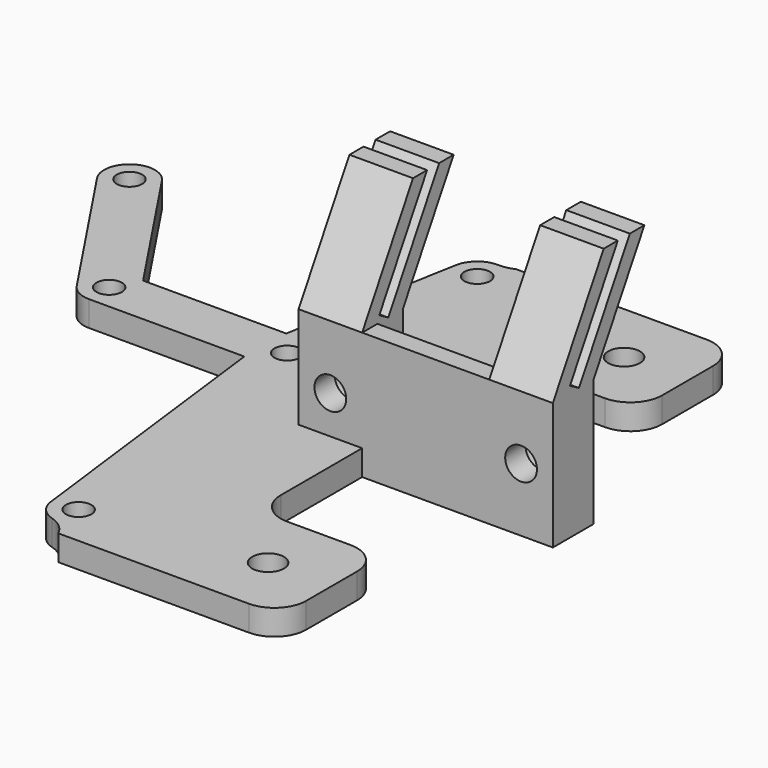
from build123d import *

# Parameters (mm, degrees)
F0_W         = 20
F0_H         = 4
F1_DEPTH     = 20
F2_DEPTH     = 20
F4_START     = 10
F4_DEPTH     = 10
F5_START     = -10
F5_DEPTH     = 10
F6_R         = 2.5
F7_DEPTH     = 25
F6_R_2       = 4.25
F8_DEPTH     = 4
F9_DEPTH     = 1
F10_W        = 20
F10_H        = 20
F10_R        = 2.5
F10_R_2      = 2
F11_DEPTH    = 4
F12_T1_DEPTH = 4
F13_R        = 5


# Not quite as in the source:
# - a fillet or chamfer that OpenCascade refuses, or shapes differently, is made with other operations: its cross-section is extruded or revolved along the edge and cut away or added
# - ends of sketch curves that miss each other by under 0.0002 mm in the source are joined


with BuildPart() as f1:
    # F0 (on Top) → F1 (new body)
    with BuildSketch(Plane.XY):
        with Locations((0, -2)):
            Rectangle(F0_W, F0_H)
    extrude(amount=F1_DEPTH)

    # F0 (on Top) → F2 (join)
    with BuildSketch(Plane.XY):
        Polygon((-10, 4), (-20, 4), (-20, -4), (-10, -4), (-10, 0), align=None)
        Polygon((20, 4), (10, 4), (10, 0), (10, -4), (20, -4), align=None)
    extrude(amount=F2_DEPTH)

    # F3 (on Right) → F4 (join)
    with BuildSketch(Plane.YZ.offset(F4_START)):
        Polygon((-4, 20), (-1.2287187079, 20), (-0.636934682, 21.025), (8.7712812921, 37.3205080757), (6, 37.3205080757), align=None)
        Polygon((-1.2287187079, 20), (1.1384173958, 20), (-0.636934682, 21.025), align=None)
        Polygon((1.1384173958, 20), (4, 20), (14, 37.3205080757), (11.1384173958, 37.3205080757), align=None)
    extrude(amount=F4_DEPTH)

    # F3 (on Right) → F5 (join)
    with BuildSketch(Plane.YZ.offset(F5_START)):
        Polygon((1.1384173958, 20), (4, 20), (14, 37.3205080757), (11.1384173958, 37.3205080757), align=None)
        Polygon((-4, 20), (-1.2287187079, 20), (-0.636934682, 21.025), (8.7712812921, 37.3205080757), (6, 37.3205080757), align=None)
        Polygon((-1.2287187079, 20), (1.1384173958, 20), (-0.636934682, 21.025), align=None)
    extrude(amount=-F5_DEPTH)

    # F6 (on face) → F7 (cut)
    with BuildSketch(Plane(origin=(0, 4, 0), x_dir=(-1, 0, 0), z_dir=(0, 1, 0))):
        with Locations((-15, 10)):
            Circle(F6_R)
        with Locations((15, 10)):
            Circle(F6_R)
    extrude(amount=-F7_DEPTH, mode=Mode.SUBTRACT)

    # F6 (on face) → F8 (cut)
    with BuildSketch(Plane(origin=(0, 4, 0), x_dir=(-1, 0, 0), z_dir=(0, 1, 0))):
        with Locations((-15, 10)):
            Circle(F6_R_2)
        with Locations((-15, 10)):
            Circle(F6_R, mode=Mode.SUBTRACT)
        with Locations((15, 10)):
            Circle(F6_R_2)
        with Locations((15, 10)):
            Circle(F6_R, mode=Mode.SUBTRACT)
    extrude(amount=-F8_DEPTH, mode=Mode.SUBTRACT)

    # F9 (cut): a face of the model
    f9_faces = [f1.faces().sort_by_distance(p)[0] for p in [
        (0, 0, 10),
    ]]
    extrude(f9_faces, amount=-F9_DEPTH, mode=Mode.SUBTRACT)


with BuildPart() as f11:
    # F10 (on Top) → F11 (new body)
    with BuildSketch(Plane.XY):
        with Locations((0, 35)):
            Rectangle(F10_W, F10_H)
        with Locations((0, 35)):
            Circle(F10_R, mode=Mode.SUBTRACT)
        with BuildLine():
            Line((-10, 25), (-10, 45))
            Line((-10, 45), (-25, 45))
            Line((-25, 45), (-25, 44.5))
            Line((-25, 44.5), (-25, 43.6224989992))
            ThreePointArc((-25, 43.6224989992), (-23.8944487245, 42.2320508076), (-23.5, 40.5))
            ThreePointArc((-23.5, 40.5), (-23.5159046021, 40.1436520514), (-23.5634919302, 39.7901378891))
            Line((-23.5634919302, 39.7901378891), (-25, 31.8240476839))
            Line((-25, 31.8240476839), (-25, 14))
            Line((-25, 14), (-25, 6))
            Line((-25, 6), (-25, -22.0868501472))
            Line((-25, -22.0868501472), (-23.0302620717, -38.0088984006))
            ThreePointArc((-23.0302620717, -38.0088984006), (-23.0075726861, -38.2539834488), (-23, -38.5))
            ThreePointArc((-23, -38.5), (-23.5358983849, -40.5), (-25, -41.9641016151))
            Line((-25, -41.9641016151), (-25, -42.5))
            Line((-25, -42.5), (-25, -45))
            Line((-25, -45), (-10, -45))
            Line((-10, -45), (-10, -25))
            Line((-10, -25), (-10, 25))
        make_face()
        with Locations((0, -35)):
            Rectangle(F10_W, F10_H)
        with Locations((0, -35)):
            Circle(F10_R, mode=Mode.SUBTRACT)
        with BuildLine():
            Line((-36.5356474045, 6), (-30.9697379283, -38.9911015994))
            ThreePointArc((-30.9697379283, -38.9911015994), (-29.9970323987, -35.8508875446), (-27, -34.5))
            Line((-27, -34.5), (-25, -34.5))
            Line((-25, -34.5), (-25, -22.0868501472))
            Line((-25, -22.0868501472), (-28.4746618739, 6))
            Line((-28.4746618739, 6), (-33, 6))
            Line((-33, 6), (-36.5356474045, 6))
        make_face()
        Polygon((-25, 6), (-25, 14), (-28.2141725332, 14), (-28.9556634317, 9.8880959261), (-28.4746618739, 6), align=None)
        with BuildLine():
            Line((-25, -34.5), (-25, -35.0358983849))
            ThreePointArc((-25, -35.0358983849), (-23.665464799, -36.29072976), (-23.0302620717, -38.0088984006))
            Line((-23.0302620717, -38.0088984006), (-25, -22.0868501472))
            Line((-25, -22.0868501472), (-25, -34.5))
        make_face()
        with BuildLine():
            ThreePointArc((-27, -34.5), (-25.9647238196, -34.6362966948), (-25, -35.0358983849))
            Line((-25, -35.0358983849), (-25, -34.5))
            Line((-25, -34.5), (-27, -34.5))
        make_face()
        with BuildLine():
            Line((-25, -38.5), (-25, -41.9641016151))
            ThreePointArc((-25, -41.9641016151), (-23.5358983849, -40.5), (-23, -38.5))
            ThreePointArc((-23, -38.5), (-23.0075726861, -38.2539834488), (-23.0302620717, -38.0088984006))
            ThreePointArc((-23.0302620717, -38.0088984006), (-23.665464799, -36.29072976), (-25, -35.0358983849))
            Line((-25, -35.0358983849), (-25, -38.5))
        make_face()
        with BuildLine():
            ThreePointArc((-27, -42.5), (-25.9647238196, -42.3637033052), (-25, -41.9641016151))
            Line((-25, -41.9641016151), (-25, -38.5))
            Line((-25, -38.5), (-25, -35.0358983849))
            ThreePointArc((-25, -35.0358983849), (-25.9647238196, -34.6362966948), (-27, -34.5))
            ThreePointArc((-27, -34.5), (-29.9970323987, -35.8508875446), (-30.9697379283, -38.9911015994))
            ThreePointArc((-30.9697379283, -38.9911015994), (-29.6491124554, -41.4970323987), (-27, -42.5))
        make_face()
        with Locations((-27, -38.5)):
            Circle(F10_R_2, mode=Mode.SUBTRACT)
        with BuildLine():
            Line((-27, -42.5), (-25, -42.5))
            Line((-25, -42.5), (-25, -41.9641016151))
            ThreePointArc((-25, -41.9641016151), (-25.9647238196, -42.3637033052), (-27, -42.5))
        make_face()
        Polygon((-25, -22.0868501472), (-25, 6), (-28.4746618739, 6), align=None)
        Polygon((-25, 14), (-25, 31.8240476839), (-28.2141725332, 14), align=None)
        with BuildLine():
            Line((-28.4746618739, 6), (-28.9556634317, 9.8880959261))
            Line((-28.9556634317, 9.8880959261), (-29.0634919302, 9.2901378891))
            ThreePointArc((-29.0634919302, 9.2901378891), (-30.4347951781, 6.9308430764), (-33, 6))
            Line((-33, 6), (-28.4746618739, 6))
        make_face()
        with BuildLine():
            ThreePointArc((-33, 6), (-35.6491124554, 7.0029676013), (-36.9697379283, 9.5088984006))
            Line((-36.9697379283, 9.5088984006), (-36.5356474045, 6))
            Line((-36.5356474045, 6), (-33, 6))
        make_face()
        with BuildLine():
            Line((-33, 14), (-36.3432041846, 14))
            Line((-36.3432041846, 14), (-36.9365077488, 10.7098620531))
            ThreePointArc((-36.9365077488, 10.7098620531), (-35.5652048219, 13.0691569236), (-33, 14))
        make_face()
        with BuildLine():
            Line((-28.2141725332, 14), (-33, 14))
            ThreePointArc((-33, 14), (-30.3508875446, 12.9970323987), (-29.0302620717, 10.4911015994))
            Line((-29.0302620717, 10.4911015994), (-28.9556634317, 9.8880959261))
            Line((-28.9556634317, 9.8880959261), (-28.2141725332, 14))
        make_face()
        with BuildLine():
            ThreePointArc((-27.5, 36.5), (-30.5691569236, 37.9347951781), (-31.4365080698, 41.2098621109))
            Line((-31.4365080698, 41.2098621109), (-36.3432041846, 14))
            Line((-36.3432041846, 14), (-33, 14))
            Line((-33, 14), (-28.2141725332, 14))
            Line((-28.2141725332, 14), (-25, 31.8240476839))
            Line((-25, 31.8240476839), (-25, 36.5))
            Line((-25, 36.5), (-27.5, 36.5))
        make_face()
        with BuildLine():
            ThreePointArc((-23.5634919302, 39.7901378891), (-24.0630881272, 38.4536283871), (-25, 37.3775010008))
            Line((-25, 37.3775010008), (-25, 36.5))
            Line((-25, 36.5), (-25, 31.8240476839))
            Line((-25, 31.8240476839), (-23.5634919302, 39.7901378891))
        make_face()
        with BuildLine():
            Line((-25, 36.5), (-25, 37.3775010008))
            ThreePointArc((-25, 37.3775010008), (-26.1752351146, 36.7257453718), (-27.5, 36.5))
            Line((-27.5, 36.5), (-25, 36.5))
        make_face()
        with BuildLine():
            Line((-25, 37.3775010008), (-25, 43.6224989992))
            ThreePointArc((-25, 43.6224989992), (-26.1752351146, 44.2742546282), (-27.5, 44.5))
            ThreePointArc((-27.5, 44.5), (-30.0652048219, 43.5691569236), (-31.4365080698, 41.2098621109))
            ThreePointArc((-31.4365080698, 41.2098621109), (-30.5691569236, 37.9347951781), (-27.5, 36.5))
            ThreePointArc((-27.5, 36.5), (-26.1752351146, 36.7257453718), (-25, 37.3775010008))
        make_face()
        with Locations((-27.5, 40.5)):
            Circle(F10_R_2, mode=Mode.SUBTRACT)
        with BuildLine():
            ThreePointArc((-23.5, 40.5), (-23.8944487245, 42.2320508076), (-25, 43.6224989992))
            Line((-25, 43.6224989992), (-25, 37.3775010008))
            ThreePointArc((-25, 37.3775010008), (-24.0630881272, 38.4536283871), (-23.5634919302, 39.7901378891))
            ThreePointArc((-23.5634919302, 39.7901378891), (-23.5159046021, 40.1436520514), (-23.5, 40.5))
        make_face()
        with BuildLine():
            Line((-25, 43.6224989992), (-25, 44.5))
            Line((-25, 44.5), (-27.5, 44.5))
            ThreePointArc((-27.5, 44.5), (-26.1752351146, 44.2742546282), (-25, 43.6224989992))
        make_face()
        with BuildLine():
            Line((-36.9365077488, 10.7098620531), (-36.3432041846, 14))
            Line((-36.3432041846, 14), (-58.859264966, 14))
            Line((-58.859264966, 14), (-57.6717988226, 12.2188007849))
            ThreePointArc((-57.6717988226, 12.2188007849), (-57.171631894, 11.1591365948), (-57, 10))
            ThreePointArc((-57, 10), (-58.1715728753, 7.1715728753), (-61, 6))
            Line((-61, 6), (-36.5356474045, 6))
            Line((-36.5356474045, 6), (-36.9697379283, 9.5088984006))
            ThreePointArc((-36.9697379283, 9.5088984006), (-36.9984696952, 10.1106349684), (-36.9365077488, 10.7098620531))
        make_face()
        with BuildLine():
            ThreePointArc((-57, 10), (-57.171631894, 11.1591365948), (-57.6717988226, 12.2188007849))
            ThreePointArc((-57.6717988226, 12.2188007849), (-59.1125682979, 13.5266983951), (-61, 14))
            ThreePointArc((-61, 14), (-64.5266983951, 11.8874317021), (-64.3282011774, 7.7811992151))
            ThreePointArc((-64.3282011774, 7.7811992151), (-62.8874317021, 6.4733016049), (-61, 6))
            ThreePointArc((-61, 6), (-58.1715728753, 7.1715728753), (-57, 10))
        make_face()
        with Locations((-61, 10)):
            Circle(F10_R_2, mode=Mode.SUBTRACT)
        with BuildLine():
            Line((-57.6717988226, 12.2188007849), (-58.859264966, 14))
            Line((-58.859264966, 14), (-61, 14))
            ThreePointArc((-61, 14), (-59.1125682979, 13.5266983951), (-57.6717988226, 12.2188007849))
        make_face()
        with BuildLine():
            Line((-61, 14), (-58.859264966, 14))
            Line((-58.859264966, 14), (-73.6717988226, 36.2188007849))
            ThreePointArc((-73.6717988226, 36.2188007849), (-73.171631894, 35.1591365948), (-73, 34))
            ThreePointArc((-73, 34), (-75.8408634052, 30.171631894), (-80.3282011774, 31.7811992151))
            Line((-80.3282011774, 31.7811992151), (-64.3282011774, 7.7811992151))
            ThreePointArc((-64.3282011774, 7.7811992151), (-64.5266983951, 11.8874317021), (-61, 14))
        make_face()
        with BuildLine():
            ThreePointArc((-73, 34), (-73.171631894, 35.1591365948), (-73.6717988226, 36.2188007849))
            ThreePointArc((-73.6717988226, 36.2188007849), (-79.2188007849, 37.3282011774), (-80.3282011774, 31.7811992151))
            ThreePointArc((-80.3282011774, 31.7811992151), (-75.8408634052, 30.171631894), (-73, 34))
        make_face()
        with Locations((-77, 34)):
            Circle(F10_R_2, mode=Mode.SUBTRACT)
        with BuildLine():
            ThreePointArc((-33, 14), (-35.5652048219, 13.0691569236), (-36.9365080698, 10.7098621109))
            ThreePointArc((-36.9365080698, 10.7098621109), (-36.9984696952, 10.1106349684), (-36.9697379283, 9.5088984006))
            ThreePointArc((-36.9697379283, 9.5088984006), (-35.6491124554, 7.0029676013), (-33, 6))
            ThreePointArc((-33, 6), (-30.4347951781, 6.9308430764), (-29.0634919302, 9.2901378891))
            ThreePointArc((-29.0634919302, 9.2901378891), (-29.0159046021, 9.6436520514), (-29, 10))
            ThreePointArc((-29, 10), (-29.0075726861, 10.2460165512), (-29.0302620717, 10.4911015994))
            ThreePointArc((-29.0302620717, 10.4911015994), (-30.3508875446, 12.9970323987), (-33, 14))
        make_face()
        with Locations((-33, 10)):
            Circle(F10_R_2, mode=Mode.SUBTRACT)
        with BuildLine():
            Line((-28.9556634317, 9.8880959261), (-29.0302620717, 10.4911015994))
            ThreePointArc((-29.0302620717, 10.4911015994), (-29.0075726861, 10.2460165512), (-29, 10))
            ThreePointArc((-29, 10), (-29.0159046021, 9.6436520514), (-29.0634919302, 9.2901378891))
            Line((-29.0634919302, 9.2901378891), (-28.9556634317, 9.8880959261))
        make_face()
    extrude(amount=F11_DEPTH)

    # F12: fillet of radius 5 on 2 edges, made by hand

    # F12_s2 → F12_t1 (join)
    with BuildSketch(Plane.XY):
        with BuildLine():
            ThreePointArc((-28.1194295133, -42.340166346), (-26.2745879363, -43.335688946), (-25, -45))
            Line((-25, -45), (-24.5481283595, -44.7859625722))
            ThreePointArc((-24.5481283595, -44.7859625722), (-24.5, -43.75), (-24.5, -42.5))
            Line((-24.5, -42.5), (-25, -42))
            ThreePointArc((-25, -42), (-27, -42), (-27.9795008241, -41.8601455527))
            Line((-27.9795008241, -41.8601455527), (-28.1194295133, -42.340166346))
        make_face()
        with BuildLine():
            ThreePointArc((-25, 45), (-26.061415483, 44.6266028276), (-27.1794494718, 44.5))
            Line((-27.1794494718, 44.5), (-25, 44.5))
            Line((-25, 44.5), (-25, 45))
        make_face()
    extrude(amount=F12_T1_DEPTH)

    # F13
    f13_edges = [f11.edges().sort_by_distance(p)[0] for p in [
        (10, 45, 2),
        (10, 25, 2),
        (-10, 25, 2),
        (-10, -25, 2),
        (10, -25, 2),
        (10, -45, 2),
    ]]
    fillet(f13_edges, radius=F13_R)


solid = Compound([f1.part, f11.part])
